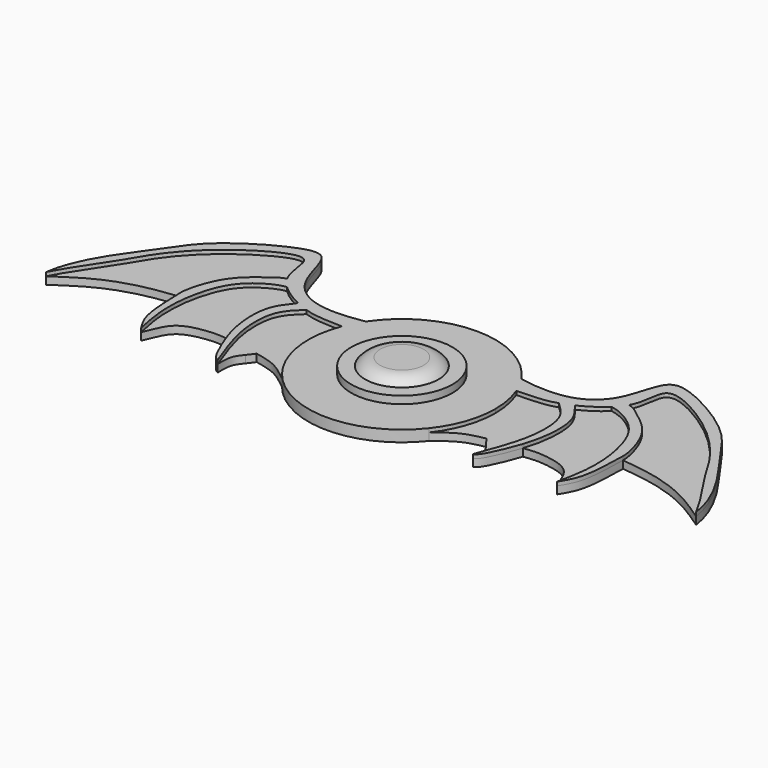
from build123d import *

# Parameters (mm, degrees)
F1_DEPTH = 3
F2_R     = 13.5064277213
F3_DEPTH = 5
F4_R     = 9.8042212389
F5_DEPTH = 7
F7_DEPTH = 2
F8_DEPTH = 3


# Not quite as in the source:
# - a fillet or chamfer that OpenCascade refuses, or shapes differently, is made with other operations: its cross-section is extruded or revolved along the edge and cut away or added


with BuildPart() as f1:
    # F0 (on Top) → F1 (new body)
    with BuildSketch(Plane.XY):
        with BuildLine():
            ThreePointArc((-19.6218875172, -15.4913372651), (0, -25), (19.6218875172, -15.4913372651))
            add(Edge.make_bspline(
                [(20.7636337812, 13.92377507), (18.884492427, 12.8973675107), (13.2694896297, 9.830391573), (17.0839746859, -5.3747888898), (19.6218875172, -15.4913372651)],
                knots=[0, 0, 0, 0, 0.3346643665, 1, 1, 1, 1], degree=3))
            ThreePointArc((20.7636337812, 13.92377507), (0, 25), (-20.7636337812, 13.92377507))
            add(Edge.make_bspline(
                [(-20.7636337812, 13.92377507), (-18.884492427, 12.8973675107), (-13.2694896297, 9.830391573), (-17.0839746859, -5.3747888898), (-19.6218875172, -15.4913372651)],
                knots=[0, 0, 0, 0, 0.3346643665, 1, 1, 1, 1], degree=3))
        make_face()
        with BuildLine():
            ThreePointArc((19.6218875172, -15.4913372651), (23.61723087, -8.1991710578), (25, 0))
            ThreePointArc((25, 0), (24.5689951544, 4.6221723357), (23.2908418319, 9.0849703775))
            ThreePointArc((23.2908418319, 9.0849703775), (22.1597092287, 11.5735598197), (20.7636337812, 13.92377507))
            add(Edge.make_bspline(
                [(20.7636337812, 13.92377507), (18.884492427, 12.8973675107), (13.2694896297, 9.830391573), (17.0839746859, -5.3747888898), (19.6218875172, -15.4913372651)],
                knots=[0, 0, 0, 0, 0.3346643665, 1, 1, 1, 1], degree=3))
        make_face()
        with BuildLine():
            ThreePointArc((-23.2908418319, 9.0849703775), (-24.7259844978, -3.6912993126), (-19.6218875172, -15.4913372651))
            add(Edge.make_bspline(
                [(-20.7636337812, 13.92377507), (-18.884492427, 12.8973675107), (-13.2694896297, 9.830391573), (-17.0839746859, -5.3747888898), (-19.6218875172, -15.4913372651)],
                knots=[0, 0, 0, 0, 0.3346643665, 1, 1, 1, 1], degree=3))
            ThreePointArc((-20.7636337812, 13.92377507), (-22.1597092287, 11.5735598197), (-23.2908418319, 9.0849703775))
        make_face()
    extrude(amount=F1_DEPTH)

    # F2 (on Top) → F3 (join)
    with BuildSketch(Plane.XY):
        Circle(F2_R)
    extrude(amount=F3_DEPTH)

    # F4 (on Top) → F5 (join)
    with BuildSketch(Plane.XY):
        Circle(F4_R)
    extrude(amount=F5_DEPTH)

    # F6: fillet of radius 5 on 1 edges, made by hand

    # F6_s1 → F6_t2 (revolve, cut)
    with BuildSketch(Plane.XZ):
        with BuildLine():
            ThreePointArc((9.8042212389, 5), (8.0402892164, 6.472135955), (5.8042212389, 7))
            Line((5.8042212389, 7), (9.8042212389, 7))
            Line((9.8042212389, 7), (9.8042212389, 5))
        make_face()
    revolve(axis=Axis((0, 0, 7), (0, 0, 1)), mode=Mode.SUBTRACT)

    # F0 (on Top) → F7 (join)
    with BuildSketch(Plane.XY):
        with BuildLine():
            ThreePointArc((20.7636337812, 13.92377507), (22.1597092287, 11.5735598197), (23.2908418319, 9.0849703775))
            add(Edge.make_bspline(
                [(23.2908418319, 9.0849703775), (27.8215143515, 9.3257680742), (30.2320226011, 9.1590800923), (33.7177366018, 10.2821364999)],
                knots=[0, 0, 0, 0, 0.1231403921, 0.1231403921, 0.1231403921, 0.1231403921], degree=3))
            add(Edge.make_bspline(
                [(33.7177366018, 10.2821364999), (34.7454077104, 10.6132401484), (35.866536795, 11.0564496893), (37.004531993, 11.5978625395)],
                knots=[0.1231403921, 0.1231403921, 0.1231403921, 0.1231403921, 0.1594450984, 0.1594450984, 0.1594450984, 0.1594450984], degree=3))
            add(Edge.make_bspline(
                [(37.004531993, 11.5978625395), (39.2474500295, 12.6649537267), (41.555886116, 14.1135251746), (43.3434300018, 15.8371345407)],
                knots=[0.1594450984, 0.1594450984, 0.1594450984, 0.1594450984, 0.2309994255, 0.2309994255, 0.2309994255, 0.2309994255], degree=3))
            add(Edge.make_bspline(
                [(43.3434300018, 15.8371345407), (44.2810928585, 16.7412603051), (45.0754287668, 17.7210645793), (45.641798526, 18.7611840665)],
                knots=[0.2309994255, 0.2309994255, 0.2309994255, 0.2309994255, 0.2685335165, 0.2685335165, 0.2685335165, 0.2685335165], degree=3))
            add(Edge.make_bspline(
                [(45.641798526, 18.7611840665), (47.3352689159, 21.8711868955), (46.777744727, 27.7747473366), (51.8560066338, 29.065553317), (66.3600577374, 20.2512677808), (74.7298542288, 9.6960609054), (77.7930462557, 3.5527051654), (84.7415977894, -6.1442317778), (86.8003591895, -10.2821364999)],
                knots=[0.2685335165, 0.2685335165, 0.2685335165, 0.2685335165, 0.3807620926, 0.4500912377, 0.6051903106, 0.7450551623, 0.8470726585, 1, 1, 1, 1], degree=3))
            add(Edge.make_bspline(
                [(20.7636337812, 13.92377507), (25.353260156, 13.083604301), (34.3722799665, 12.4739559617), (43.1666874947, 19.3658325346), (44.7883389447, 31.8865702273), (51.6235191398, 32.3410311281), (68.757647719, 22.5890249267), (75.2339965242, 11.4273433149), (85.5971213344, -1.5157287213), (86.8003591895, -10.2821364999)],
                knots=[0, 0, 0, 0, 0.1438051462, 0.2702269745, 0.4006587664, 0.4888335416, 0.6586500337, 0.8053535671, 1, 1, 1, 1], degree=3))
        make_face()
        with BuildLine():
            ThreePointArc((19.6218875172, -15.4913372651), (23.61723087, -8.1991710578), (25, 0))
            ThreePointArc((25, 0), (24.5689951544, 4.6221723357), (23.2908418319, 9.0849703775))
            ThreePointArc((23.2908418319, 9.0849703775), (22.1597092287, 11.5735598197), (20.7636337812, 13.92377507))
            add(Edge.make_bspline(
                [(20.7636337812, 13.92377507), (18.884492427, 12.8973675107), (13.2694896297, 9.830391573), (17.0839746859, -5.3747888898), (19.6218875172, -15.4913372651)],
                knots=[0, 0, 0, 0, 0.3346643665, 1, 1, 1, 1], degree=3))
        make_face()
        with BuildLine():
            ThreePointArc((23.2908418319, 9.0849703775), (24.5689951544, 4.6221723357), (25, 0))
            ThreePointArc((25, 0), (23.61723087, -8.1991710578), (19.6218875172, -15.4913372651))
            add(Edge.make_bspline(
                [(19.6218875172, -15.4913372651), (21.4152102231, -14.0609489213), (24.8604058768, -11.2746200768), (28.7928801922, -10.5001506768), (30.6888949126, -10.1227229461)],
                knots=[0, 0, 0, 0, 0.5172233423, 1, 1, 1, 1], degree=3))
            add(Edge.make_bspline(
                [(32.1116161516, -12.0142660523), (31.6373757386, -11.3837516835), (31.1631353256, -10.7532373148), (30.6888949126, -10.1227229461)],
                knots=[0, 0, 0, 0, 2.3668694612, 2.3668694612, 2.3668694612, 2.3668694612], degree=3))
            add(Edge.make_bspline(
                [(32.1116161516, -12.0142660523), (32.776720922, -12.8822985255), (34.1447409362, -14.3321949992), (34.1047637318, -17.2769145921), (34.0780636316, -18.8904348761)],
                knots=[0, 0, 0, 0, 0.4499025437, 1, 1, 1, 1], degree=3))
            add(Edge.make_bspline(
                [(33.7177366018, 10.2821364999), (35.3645415529, 8.7757476619), (38.884943387, 5.4848056386), (38.8140830901, -4.1284440887), (37.0736184249, -10.5819579136), (35.282158389, -15.8523198225), (34.0780636316, -18.8904348761)],
                knots=[0, 0, 0, 0, 0.2318500383, 0.4998701646, 0.7334854658, 1, 1, 1, 1], degree=3))
            add(Edge.make_bspline(
                [(23.2908418319, 9.0849703775), (27.8215143515, 9.3257680742), (30.2320226011, 9.1590800923), (33.7177366018, 10.2821364999)],
                knots=[0, 0, 0, 0, 0.1231403921, 0.1231403921, 0.1231403921, 0.1231403921], degree=3))
        make_face()
        with BuildLine():
            add(Edge.make_bspline(
                [(33.7177366018, 10.2821364999), (34.7454077104, 10.6132401484), (35.866536795, 11.0564496893), (37.004531993, 11.5978625395)],
                knots=[0.1231403921, 0.1231403921, 0.1231403921, 0.1231403921, 0.1594450984, 0.1594450984, 0.1594450984, 0.1594450984], degree=3))
            add(Edge.make_bspline(
                [(33.7177366018, 10.2821364999), (35.3645415529, 8.7757476619), (38.884943387, 5.4848056386), (38.8140830901, -4.1284440887), (37.0736184249, -10.5819579136), (35.282158389, -15.8523198225), (34.0780636316, -18.8904348761)],
                knots=[0, 0, 0, 0, 0.2318500383, 0.4998701646, 0.7334854658, 1, 1, 1, 1], degree=3))
            add(Edge.make_bspline(
                [(39.3599004471, -8.7854920866), (38.7249404903, -10.7452749087), (37.0180617267, -14.9012626381), (35.2493275964, -18.5335928874), (34.0780636316, -18.8904348761)],
                knots=[0.6277129418, 0.6277129418, 0.6277129418, 0.6277129418, 0.792816444, 1, 1, 1, 1], degree=3))
            add(Edge.make_bspline(
                [(37.004531993, 11.5978625395), (38.0800679502, 10.0046793736), (41.3336069296, 6.7268291074), (41.1834657071, -2.2502985215), (39.8295408824, -7.3359624778), (39.3599004471, -8.7854920866)],
                knots=[0, 0, 0, 0, 0.2173363693, 0.5055961378, 0.6277129418, 0.6277129418, 0.6277129418, 0.6277129418], degree=3))
        make_face()
        with BuildLine():
            add(Edge.make_bspline(
                [(37.004531993, 11.5978625395), (39.2474500295, 12.6649537267), (41.555886116, 14.1135251746), (43.3434300018, 15.8371345407)],
                knots=[0.1594450984, 0.1594450984, 0.1594450984, 0.1594450984, 0.2309994255, 0.2309994255, 0.2309994255, 0.2309994255], degree=3))
            add(Edge.make_bspline(
                [(37.004531993, 11.5978625395), (38.0800679502, 10.0046793736), (41.3336069296, 6.7268291074), (41.1834657071, -2.2502985215), (39.8295408824, -7.3359624778), (39.3599004471, -8.7854920866)],
                knots=[0, 0, 0, 0, 0.2173363693, 0.5055961378, 0.6277129418, 0.6277129418, 0.6277129418, 0.6277129418], degree=3))
            add(Edge.make_bspline(
                [(55.5573105812, -17.6151320338), (54.4439075888, -14.9875635555), (52.9703835571, -10.411043477), (46.6717355198, -8.6507292972), (42.2245726074, -8.3797506367), (40.2332096515, -8.6600986878), (39.3599004471, -8.7854920866)],
                knots=[0, 0, 0, 0, 0.3047383368, 0.5764576192, 0.8133522424, 1, 1, 1, 1], degree=3))
            add(Edge.make_bspline(
                [(43.3434300018, 15.8371345407), (45.3565623966, 15.5676262825), (49.9854795603, 13.2408710445), (54.5376514308, 8.1613285539), (57.1013516863, -1.3778788699), (57.1238501467, -10.2186225385), (56.0702038202, -15.2273425566), (55.5573105812, -17.6151320338)],
                knots=[0, 0, 0, 0, 0.1860076727, 0.3714288806, 0.5926344587, 0.8055769314, 1, 1, 1, 1], degree=3))
        make_face()
        with BuildLine():
            add(Edge.make_bspline(
                [(45.641798526, 18.7611840665), (47.0236524725, 18.4958354205), (50.5733406235, 15.7663353525), (56.3104736797, 11.1079119823), (58.8622688049, 3.2726876511), (59.0809752339, 0.6245344364), (59.0938226065, 0)],
                knots=[0, 0, 0, 0, 0.146943127, 0.3231645985, 0.5131967694, 0.5724247553, 0.5724247553, 0.5724247553, 0.5724247553], degree=3))
            add(Edge.make_bspline(
                [(43.3434300018, 15.8371345407), (44.2810928585, 16.7412603051), (45.0754287668, 17.7210645793), (45.641798526, 18.7611840665)],
                knots=[0.2309994255, 0.2309994255, 0.2309994255, 0.2309994255, 0.2685335165, 0.2685335165, 0.2685335165, 0.2685335165], degree=3))
            add(Edge.make_bspline(
                [(43.3434300018, 15.8371345407), (45.3565623966, 15.5676262825), (49.9854795603, 13.2408710445), (54.5376514308, 8.1613285539), (57.1013516863, -1.3778788699), (57.1238501467, -10.2186225385), (56.0702038202, -15.2273425566), (55.5573105812, -17.6151320338)],
                knots=[0, 0, 0, 0, 0.1860076727, 0.3714288806, 0.5926344587, 0.8055769314, 1, 1, 1, 1], degree=3))
            add(Edge.make_bspline(
                [(59.0938226065, 0), (59.1104927586, -0.8103667818), (58.9358631638, -3.6588287886), (58.782367202, -12.4944121501), (56.5431938855, -16.0569735079), (55.5573105812, -17.6151320338)],
                knots=[0.5724247553, 0.5724247553, 0.5724247553, 0.5724247553, 0.6492762299, 0.8452276156, 1, 1, 1, 1], degree=3))
        make_face()
        with BuildLine():
            add(Edge.make_bspline(
                [(59.0938226065, 0), (62.0265888913, -0.341290779), (68.0943487487, -1.0474058551), (78.0033682979, -4.2880779786), (83.850491985, -8.272167765), (86.8003591895, -10.2821364999)],
                knots=[0, 0, 0, 0, 0.3167243267, 0.6552882052, 1, 1, 1, 1], degree=3))
            add(Edge.make_bspline(
                [(45.641798526, 18.7611840665), (47.3352689159, 21.8711868955), (46.777744727, 27.7747473366), (51.8560066338, 29.065553317), (66.3600577374, 20.2512677808), (74.7298542288, 9.6960609054), (77.7930462557, 3.5527051654), (84.7415977894, -6.1442317778), (86.8003591895, -10.2821364999)],
                knots=[0.2685335165, 0.2685335165, 0.2685335165, 0.2685335165, 0.3807620926, 0.4500912377, 0.6051903106, 0.7450551623, 0.8470726585, 1, 1, 1, 1], degree=3))
            add(Edge.make_bspline(
                [(45.641798526, 18.7611840665), (47.0236524725, 18.4958354205), (50.5733406235, 15.7663353525), (56.3104736797, 11.1079119823), (58.8622688049, 3.2726876511), (59.0809752339, 0.6245344364), (59.0938226065, 0)],
                knots=[0, 0, 0, 0, 0.146943127, 0.3231645985, 0.5131967694, 0.5724247553, 0.5724247553, 0.5724247553, 0.5724247553], degree=3))
        make_face()
        with BuildLine():
            add(Edge.make_bspline(
                [(-19.6218875172, -15.4913372651), (-21.4152102231, -14.0609489213), (-24.8604058768, -11.2746200768), (-28.7928801922, -10.5001506768), (-30.6888949126, -10.1227229461)],
                knots=[0, 0, 0, 0, 0.5172233423, 1, 1, 1, 1], degree=3))
            ThreePointArc((-19.6218875172, -15.4913372651), (-24.7259844978, -3.6912993126), (-23.2908418319, 9.0849703775))
            add(Edge.make_bspline(
                [(-23.2908418319, 9.0849703775), (-27.8215143515, 9.3257680742), (-30.2320226011, 9.1590800923), (-33.7177366018, 10.2821364999)],
                knots=[0, 0, 0, 0, 0.1231403921, 0.1231403921, 0.1231403921, 0.1231403921], degree=3))
            add(Edge.make_bspline(
                [(-33.7177366018, 10.2821364999), (-35.3645415529, 8.7757476619), (-38.884943387, 5.4848056386), (-38.8140830901, -4.1284440887), (-37.0736184249, -10.5819579136), (-35.282158389, -15.8523198225), (-34.0780636316, -18.8904348761)],
                knots=[0, 0, 0, 0, 0.2318500383, 0.4998701646, 0.7334854658, 1, 1, 1, 1], degree=3))
            add(Edge.make_bspline(
                [(-32.1116161516, -12.0142660523), (-32.776720922, -12.8822985255), (-34.1447409362, -14.3321949992), (-34.1047637318, -17.2769145921), (-34.0780636316, -18.8904348761)],
                knots=[0, 0, 0, 0, 0.4499025437, 1, 1, 1, 1], degree=3))
            add(Edge.make_bspline(
                [(-32.1116161516, -12.0142660523), (-31.6373757386, -11.3837516835), (-31.1631353256, -10.7532373148), (-30.6888949126, -10.1227229461)],
                knots=[0, 0, 0, 0, 2.3668694612, 2.3668694612, 2.3668694612, 2.3668694612], degree=3))
        make_face()
        with BuildLine():
            add(Edge.make_bspline(
                [(-37.004531993, 11.5978625395), (-38.0800679502, 10.0046793736), (-41.3336069296, 6.7268291074), (-41.1834657071, -2.2502985215), (-39.8295408824, -7.3359624778), (-39.3599004471, -8.7854920866)],
                knots=[0, 0, 0, 0, 0.2173363693, 0.5055961378, 0.6277129418, 0.6277129418, 0.6277129418, 0.6277129418], degree=3))
            add(Edge.make_bspline(
                [(-37.004531993, 11.5978625395), (-39.2474500295, 12.6649537267), (-41.555886116, 14.1135251746), (-43.3434300018, 15.8371345407)],
                knots=[0.1594450984, 0.1594450984, 0.1594450984, 0.1594450984, 0.2309994255, 0.2309994255, 0.2309994255, 0.2309994255], degree=3))
            add(Edge.make_bspline(
                [(-43.3434300018, 15.8371345407), (-45.3565623966, 15.5676262825), (-49.9854795603, 13.2408710445), (-54.5376514308, 8.1613285539), (-57.1013516863, -1.3778788699), (-57.1238501467, -10.2186225385), (-56.0702038202, -15.2273425566), (-55.5573105812, -17.6151320338)],
                knots=[0, 0, 0, 0, 0.1860076727, 0.3714288806, 0.5926344587, 0.8055769314, 1, 1, 1, 1], degree=3))
            add(Edge.make_bspline(
                [(-55.5573105812, -17.6151320338), (-54.4439075888, -14.9875635555), (-52.9703835571, -10.411043477), (-46.6717355198, -8.6507292972), (-42.2245726074, -8.3797506367), (-40.2332096515, -8.6600986878), (-39.3599004471, -8.7854920866)],
                knots=[0, 0, 0, 0, 0.3047383368, 0.5764576192, 0.8133522424, 1, 1, 1, 1], degree=3))
        make_face()
        with BuildLine():
            add(Edge.make_bspline(
                [(-33.7177366018, 10.2821364999), (-35.3645415529, 8.7757476619), (-38.884943387, 5.4848056386), (-38.8140830901, -4.1284440887), (-37.0736184249, -10.5819579136), (-35.282158389, -15.8523198225), (-34.0780636316, -18.8904348761)],
                knots=[0, 0, 0, 0, 0.2318500383, 0.4998701646, 0.7334854658, 1, 1, 1, 1], degree=3))
            add(Edge.make_bspline(
                [(-33.7177366018, 10.2821364999), (-34.7454077104, 10.6132401484), (-35.866536795, 11.0564496893), (-37.004531993, 11.5978625395)],
                knots=[0.1231403921, 0.1231403921, 0.1231403921, 0.1231403921, 0.1594450984, 0.1594450984, 0.1594450984, 0.1594450984], degree=3))
            add(Edge.make_bspline(
                [(-37.004531993, 11.5978625395), (-38.0800679502, 10.0046793736), (-41.3336069296, 6.7268291074), (-41.1834657071, -2.2502985215), (-39.8295408824, -7.3359624778), (-39.3599004471, -8.7854920866)],
                knots=[0, 0, 0, 0, 0.2173363693, 0.5055961378, 0.6277129418, 0.6277129418, 0.6277129418, 0.6277129418], degree=3))
            add(Edge.make_bspline(
                [(-39.3599004471, -8.7854920866), (-38.7249404903, -10.7452749087), (-37.0180617267, -14.9012626381), (-35.2493275964, -18.5335928874), (-34.0780636316, -18.8904348761)],
                knots=[0.6277129418, 0.6277129418, 0.6277129418, 0.6277129418, 0.792816444, 1, 1, 1, 1], degree=3))
        make_face()
        with BuildLine():
            ThreePointArc((-23.2908418319, 9.0849703775), (-22.1597092287, 11.5735598197), (-20.7636337812, 13.92377507))
            add(Edge.make_bspline(
                [(-20.7636337812, 13.92377507), (-25.353260156, 13.083604301), (-34.3722799665, 12.4739559617), (-43.1666874947, 19.3658325346), (-44.7883389447, 31.8865702273), (-51.6235191398, 32.3410311281), (-68.757647719, 22.5890249267), (-75.2339965242, 11.4273433149), (-85.5971213344, -1.5157287213), (-86.8003591895, -10.2821364999)],
                knots=[0, 0, 0, 0, 0.1438051462, 0.2702269745, 0.4006587664, 0.4888335416, 0.6586500337, 0.8053535671, 1, 1, 1, 1], degree=3))
            add(Edge.make_bspline(
                [(-45.641798526, 18.7611840665), (-47.3352689159, 21.8711868955), (-46.777744727, 27.7747473366), (-51.8560066338, 29.065553317), (-66.3600577374, 20.2512677808), (-74.7298542288, 9.6960609054), (-77.7930462557, 3.5527051654), (-84.7415977894, -6.1442317778), (-86.8003591895, -10.2821364999)],
                knots=[0.2685335165, 0.2685335165, 0.2685335165, 0.2685335165, 0.3807620926, 0.4500912377, 0.6051903106, 0.7450551623, 0.8470726585, 1, 1, 1, 1], degree=3))
            add(Edge.make_bspline(
                [(-43.3434300018, 15.8371345407), (-44.2810928585, 16.7412603051), (-45.0754287668, 17.7210645793), (-45.641798526, 18.7611840665)],
                knots=[0.2309994255, 0.2309994255, 0.2309994255, 0.2309994255, 0.2685335165, 0.2685335165, 0.2685335165, 0.2685335165], degree=3))
            add(Edge.make_bspline(
                [(-37.004531993, 11.5978625395), (-39.2474500295, 12.6649537267), (-41.555886116, 14.1135251746), (-43.3434300018, 15.8371345407)],
                knots=[0.1594450984, 0.1594450984, 0.1594450984, 0.1594450984, 0.2309994255, 0.2309994255, 0.2309994255, 0.2309994255], degree=3))
            add(Edge.make_bspline(
                [(-33.7177366018, 10.2821364999), (-34.7454077104, 10.6132401484), (-35.866536795, 11.0564496893), (-37.004531993, 11.5978625395)],
                knots=[0.1231403921, 0.1231403921, 0.1231403921, 0.1231403921, 0.1594450984, 0.1594450984, 0.1594450984, 0.1594450984], degree=3))
            add(Edge.make_bspline(
                [(-23.2908418319, 9.0849703775), (-27.8215143515, 9.3257680742), (-30.2320226011, 9.1590800923), (-33.7177366018, 10.2821364999)],
                knots=[0, 0, 0, 0, 0.1231403921, 0.1231403921, 0.1231403921, 0.1231403921], degree=3))
        make_face()
        with BuildLine():
            add(Edge.make_bspline(
                [(-45.641798526, 18.7611840665), (-47.3352689159, 21.8711868955), (-46.777744727, 27.7747473366), (-51.8560066338, 29.065553317), (-66.3600577374, 20.2512677808), (-74.7298542288, 9.6960609054), (-77.7930462557, 3.5527051654), (-84.7415977894, -6.1442317778), (-86.8003591895, -10.2821364999)],
                knots=[0.2685335165, 0.2685335165, 0.2685335165, 0.2685335165, 0.3807620926, 0.4500912377, 0.6051903106, 0.7450551623, 0.8470726585, 1, 1, 1, 1], degree=3))
            add(Edge.make_bspline(
                [(-59.0938226065, 0), (-62.0265888913, -0.341290779), (-68.0943487487, -1.0474058551), (-78.0033682979, -4.2880779786), (-83.850491985, -8.272167765), (-86.8003591895, -10.2821364999)],
                knots=[0, 0, 0, 0, 0.3167243267, 0.6552882052, 1, 1, 1, 1], degree=3))
            add(Edge.make_bspline(
                [(-45.641798526, 18.7611840665), (-47.0236524725, 18.4958354205), (-50.5733406235, 15.7663353525), (-56.3104736797, 11.1079119823), (-58.8622688049, 3.2726876511), (-59.0809752339, 0.6245344364), (-59.0938226065, 0)],
                knots=[0, 0, 0, 0, 0.146943127, 0.3231645985, 0.5131967694, 0.5724247553, 0.5724247553, 0.5724247553, 0.5724247553], degree=3))
        make_face()
        with BuildLine():
            add(Edge.make_bspline(
                [(-43.3434300018, 15.8371345407), (-44.2810928585, 16.7412603051), (-45.0754287668, 17.7210645793), (-45.641798526, 18.7611840665)],
                knots=[0.2309994255, 0.2309994255, 0.2309994255, 0.2309994255, 0.2685335165, 0.2685335165, 0.2685335165, 0.2685335165], degree=3))
            add(Edge.make_bspline(
                [(-45.641798526, 18.7611840665), (-47.0236524725, 18.4958354205), (-50.5733406235, 15.7663353525), (-56.3104736797, 11.1079119823), (-58.8622688049, 3.2726876511), (-59.0809752339, 0.6245344364), (-59.0938226065, 0)],
                knots=[0, 0, 0, 0, 0.146943127, 0.3231645985, 0.5131967694, 0.5724247553, 0.5724247553, 0.5724247553, 0.5724247553], degree=3))
            add(Edge.make_bspline(
                [(-59.0938226065, 0), (-59.1104927586, -0.8103667818), (-58.9358631638, -3.6588287886), (-58.782367202, -12.4944121501), (-56.5431938855, -16.0569735079), (-55.5573105812, -17.6151320338)],
                knots=[0.5724247553, 0.5724247553, 0.5724247553, 0.5724247553, 0.6492762299, 0.8452276156, 1, 1, 1, 1], degree=3))
            add(Edge.make_bspline(
                [(-43.3434300018, 15.8371345407), (-45.3565623966, 15.5676262825), (-49.9854795603, 13.2408710445), (-54.5376514308, 8.1613285539), (-57.1013516863, -1.3778788699), (-57.1238501467, -10.2186225385), (-56.0702038202, -15.2273425566), (-55.5573105812, -17.6151320338)],
                knots=[0, 0, 0, 0, 0.1860076727, 0.3714288806, 0.5926344587, 0.8055769314, 1, 1, 1, 1], degree=3))
        make_face()
        with BuildLine():
            ThreePointArc((-23.2908418319, 9.0849703775), (-24.7259844978, -3.6912993126), (-19.6218875172, -15.4913372651))
            add(Edge.make_bspline(
                [(-20.7636337812, 13.92377507), (-18.884492427, 12.8973675107), (-13.2694896297, 9.830391573), (-17.0839746859, -5.3747888898), (-19.6218875172, -15.4913372651)],
                knots=[0, 0, 0, 0, 0.3346643665, 1, 1, 1, 1], degree=3))
            ThreePointArc((-20.7636337812, 13.92377507), (-22.1597092287, 11.5735598197), (-23.2908418319, 9.0849703775))
        make_face()
    extrude(amount=F7_DEPTH)

    # F0 (on Top) → F8 (join)
    with BuildSketch(Plane.XY):
        with BuildLine():
            ThreePointArc((20.7636337812, 13.92377507), (22.1597092287, 11.5735598197), (23.2908418319, 9.0849703775))
            add(Edge.make_bspline(
                [(23.2908418319, 9.0849703775), (27.8215143515, 9.3257680742), (30.2320226011, 9.1590800923), (33.7177366018, 10.2821364999)],
                knots=[0, 0, 0, 0, 0.1231403921, 0.1231403921, 0.1231403921, 0.1231403921], degree=3))
            add(Edge.make_bspline(
                [(33.7177366018, 10.2821364999), (34.7454077104, 10.6132401484), (35.866536795, 11.0564496893), (37.004531993, 11.5978625395)],
                knots=[0.1231403921, 0.1231403921, 0.1231403921, 0.1231403921, 0.1594450984, 0.1594450984, 0.1594450984, 0.1594450984], degree=3))
            add(Edge.make_bspline(
                [(37.004531993, 11.5978625395), (39.2474500295, 12.6649537267), (41.555886116, 14.1135251746), (43.3434300018, 15.8371345407)],
                knots=[0.1594450984, 0.1594450984, 0.1594450984, 0.1594450984, 0.2309994255, 0.2309994255, 0.2309994255, 0.2309994255], degree=3))
            add(Edge.make_bspline(
                [(43.3434300018, 15.8371345407), (44.2810928585, 16.7412603051), (45.0754287668, 17.7210645793), (45.641798526, 18.7611840665)],
                knots=[0.2309994255, 0.2309994255, 0.2309994255, 0.2309994255, 0.2685335165, 0.2685335165, 0.2685335165, 0.2685335165], degree=3))
            add(Edge.make_bspline(
                [(45.641798526, 18.7611840665), (47.3352689159, 21.8711868955), (46.777744727, 27.7747473366), (51.8560066338, 29.065553317), (66.3600577374, 20.2512677808), (74.7298542288, 9.6960609054), (77.7930462557, 3.5527051654), (84.7415977894, -6.1442317778), (86.8003591895, -10.2821364999)],
                knots=[0.2685335165, 0.2685335165, 0.2685335165, 0.2685335165, 0.3807620926, 0.4500912377, 0.6051903106, 0.7450551623, 0.8470726585, 1, 1, 1, 1], degree=3))
            add(Edge.make_bspline(
                [(20.7636337812, 13.92377507), (25.353260156, 13.083604301), (34.3722799665, 12.4739559617), (43.1666874947, 19.3658325346), (44.7883389447, 31.8865702273), (51.6235191398, 32.3410311281), (68.757647719, 22.5890249267), (75.2339965242, 11.4273433149), (85.5971213344, -1.5157287213), (86.8003591895, -10.2821364999)],
                knots=[0, 0, 0, 0, 0.1438051462, 0.2702269745, 0.4006587664, 0.4888335416, 0.6586500337, 0.8053535671, 1, 1, 1, 1], degree=3))
        make_face()
        with BuildLine():
            add(Edge.make_bspline(
                [(33.7177366018, 10.2821364999), (34.7454077104, 10.6132401484), (35.866536795, 11.0564496893), (37.004531993, 11.5978625395)],
                knots=[0.1231403921, 0.1231403921, 0.1231403921, 0.1231403921, 0.1594450984, 0.1594450984, 0.1594450984, 0.1594450984], degree=3))
            add(Edge.make_bspline(
                [(33.7177366018, 10.2821364999), (35.3645415529, 8.7757476619), (38.884943387, 5.4848056386), (38.8140830901, -4.1284440887), (37.0736184249, -10.5819579136), (35.282158389, -15.8523198225), (34.0780636316, -18.8904348761)],
                knots=[0, 0, 0, 0, 0.2318500383, 0.4998701646, 0.7334854658, 1, 1, 1, 1], degree=3))
            add(Edge.make_bspline(
                [(39.3599004471, -8.7854920866), (38.7249404903, -10.7452749087), (37.0180617267, -14.9012626381), (35.2493275964, -18.5335928874), (34.0780636316, -18.8904348761)],
                knots=[0.6277129418, 0.6277129418, 0.6277129418, 0.6277129418, 0.792816444, 1, 1, 1, 1], degree=3))
            add(Edge.make_bspline(
                [(37.004531993, 11.5978625395), (38.0800679502, 10.0046793736), (41.3336069296, 6.7268291074), (41.1834657071, -2.2502985215), (39.8295408824, -7.3359624778), (39.3599004471, -8.7854920866)],
                knots=[0, 0, 0, 0, 0.2173363693, 0.5055961378, 0.6277129418, 0.6277129418, 0.6277129418, 0.6277129418], degree=3))
        make_face()
        with BuildLine():
            add(Edge.make_bspline(
                [(45.641798526, 18.7611840665), (47.0236524725, 18.4958354205), (50.5733406235, 15.7663353525), (56.3104736797, 11.1079119823), (58.8622688049, 3.2726876511), (59.0809752339, 0.6245344364), (59.0938226065, 0)],
                knots=[0, 0, 0, 0, 0.146943127, 0.3231645985, 0.5131967694, 0.5724247553, 0.5724247553, 0.5724247553, 0.5724247553], degree=3))
            add(Edge.make_bspline(
                [(43.3434300018, 15.8371345407), (44.2810928585, 16.7412603051), (45.0754287668, 17.7210645793), (45.641798526, 18.7611840665)],
                knots=[0.2309994255, 0.2309994255, 0.2309994255, 0.2309994255, 0.2685335165, 0.2685335165, 0.2685335165, 0.2685335165], degree=3))
            add(Edge.make_bspline(
                [(43.3434300018, 15.8371345407), (45.3565623966, 15.5676262825), (49.9854795603, 13.2408710445), (54.5376514308, 8.1613285539), (57.1013516863, -1.3778788699), (57.1238501467, -10.2186225385), (56.0702038202, -15.2273425566), (55.5573105812, -17.6151320338)],
                knots=[0, 0, 0, 0, 0.1860076727, 0.3714288806, 0.5926344587, 0.8055769314, 1, 1, 1, 1], degree=3))
            add(Edge.make_bspline(
                [(59.0938226065, 0), (59.1104927586, -0.8103667818), (58.9358631638, -3.6588287886), (58.782367202, -12.4944121501), (56.5431938855, -16.0569735079), (55.5573105812, -17.6151320338)],
                knots=[0.5724247553, 0.5724247553, 0.5724247553, 0.5724247553, 0.6492762299, 0.8452276156, 1, 1, 1, 1], degree=3))
        make_face()
        with BuildLine():
            ThreePointArc((-23.2908418319, 9.0849703775), (-22.1597092287, 11.5735598197), (-20.7636337812, 13.92377507))
            add(Edge.make_bspline(
                [(-20.7636337812, 13.92377507), (-25.353260156, 13.083604301), (-34.3722799665, 12.4739559617), (-43.1666874947, 19.3658325346), (-44.7883389447, 31.8865702273), (-51.6235191398, 32.3410311281), (-68.757647719, 22.5890249267), (-75.2339965242, 11.4273433149), (-85.5971213344, -1.5157287213), (-86.8003591895, -10.2821364999)],
                knots=[0, 0, 0, 0, 0.1438051462, 0.2702269745, 0.4006587664, 0.4888335416, 0.6586500337, 0.8053535671, 1, 1, 1, 1], degree=3))
            add(Edge.make_bspline(
                [(-45.641798526, 18.7611840665), (-47.3352689159, 21.8711868955), (-46.777744727, 27.7747473366), (-51.8560066338, 29.065553317), (-66.3600577374, 20.2512677808), (-74.7298542288, 9.6960609054), (-77.7930462557, 3.5527051654), (-84.7415977894, -6.1442317778), (-86.8003591895, -10.2821364999)],
                knots=[0.2685335165, 0.2685335165, 0.2685335165, 0.2685335165, 0.3807620926, 0.4500912377, 0.6051903106, 0.7450551623, 0.8470726585, 1, 1, 1, 1], degree=3))
            add(Edge.make_bspline(
                [(-43.3434300018, 15.8371345407), (-44.2810928585, 16.7412603051), (-45.0754287668, 17.7210645793), (-45.641798526, 18.7611840665)],
                knots=[0.2309994255, 0.2309994255, 0.2309994255, 0.2309994255, 0.2685335165, 0.2685335165, 0.2685335165, 0.2685335165], degree=3))
            add(Edge.make_bspline(
                [(-37.004531993, 11.5978625395), (-39.2474500295, 12.6649537267), (-41.555886116, 14.1135251746), (-43.3434300018, 15.8371345407)],
                knots=[0.1594450984, 0.1594450984, 0.1594450984, 0.1594450984, 0.2309994255, 0.2309994255, 0.2309994255, 0.2309994255], degree=3))
            add(Edge.make_bspline(
                [(-33.7177366018, 10.2821364999), (-34.7454077104, 10.6132401484), (-35.866536795, 11.0564496893), (-37.004531993, 11.5978625395)],
                knots=[0.1231403921, 0.1231403921, 0.1231403921, 0.1231403921, 0.1594450984, 0.1594450984, 0.1594450984, 0.1594450984], degree=3))
            add(Edge.make_bspline(
                [(-23.2908418319, 9.0849703775), (-27.8215143515, 9.3257680742), (-30.2320226011, 9.1590800923), (-33.7177366018, 10.2821364999)],
                knots=[0, 0, 0, 0, 0.1231403921, 0.1231403921, 0.1231403921, 0.1231403921], degree=3))
        make_face()
        with BuildLine():
            add(Edge.make_bspline(
                [(-33.7177366018, 10.2821364999), (-35.3645415529, 8.7757476619), (-38.884943387, 5.4848056386), (-38.8140830901, -4.1284440887), (-37.0736184249, -10.5819579136), (-35.282158389, -15.8523198225), (-34.0780636316, -18.8904348761)],
                knots=[0, 0, 0, 0, 0.2318500383, 0.4998701646, 0.7334854658, 1, 1, 1, 1], degree=3))
            add(Edge.make_bspline(
                [(-33.7177366018, 10.2821364999), (-34.7454077104, 10.6132401484), (-35.866536795, 11.0564496893), (-37.004531993, 11.5978625395)],
                knots=[0.1231403921, 0.1231403921, 0.1231403921, 0.1231403921, 0.1594450984, 0.1594450984, 0.1594450984, 0.1594450984], degree=3))
            add(Edge.make_bspline(
                [(-37.004531993, 11.5978625395), (-38.0800679502, 10.0046793736), (-41.3336069296, 6.7268291074), (-41.1834657071, -2.2502985215), (-39.8295408824, -7.3359624778), (-39.3599004471, -8.7854920866)],
                knots=[0, 0, 0, 0, 0.2173363693, 0.5055961378, 0.6277129418, 0.6277129418, 0.6277129418, 0.6277129418], degree=3))
            add(Edge.make_bspline(
                [(-39.3599004471, -8.7854920866), (-38.7249404903, -10.7452749087), (-37.0180617267, -14.9012626381), (-35.2493275964, -18.5335928874), (-34.0780636316, -18.8904348761)],
                knots=[0.6277129418, 0.6277129418, 0.6277129418, 0.6277129418, 0.792816444, 1, 1, 1, 1], degree=3))
        make_face()
        with BuildLine():
            add(Edge.make_bspline(
                [(-43.3434300018, 15.8371345407), (-44.2810928585, 16.7412603051), (-45.0754287668, 17.7210645793), (-45.641798526, 18.7611840665)],
                knots=[0.2309994255, 0.2309994255, 0.2309994255, 0.2309994255, 0.2685335165, 0.2685335165, 0.2685335165, 0.2685335165], degree=3))
            add(Edge.make_bspline(
                [(-45.641798526, 18.7611840665), (-47.0236524725, 18.4958354205), (-50.5733406235, 15.7663353525), (-56.3104736797, 11.1079119823), (-58.8622688049, 3.2726876511), (-59.0809752339, 0.6245344364), (-59.0938226065, 0)],
                knots=[0, 0, 0, 0, 0.146943127, 0.3231645985, 0.5131967694, 0.5724247553, 0.5724247553, 0.5724247553, 0.5724247553], degree=3))
            add(Edge.make_bspline(
                [(-59.0938226065, 0), (-59.1104927586, -0.8103667818), (-58.9358631638, -3.6588287886), (-58.782367202, -12.4944121501), (-56.5431938855, -16.0569735079), (-55.5573105812, -17.6151320338)],
                knots=[0.5724247553, 0.5724247553, 0.5724247553, 0.5724247553, 0.6492762299, 0.8452276156, 1, 1, 1, 1], degree=3))
            add(Edge.make_bspline(
                [(-43.3434300018, 15.8371345407), (-45.3565623966, 15.5676262825), (-49.9854795603, 13.2408710445), (-54.5376514308, 8.1613285539), (-57.1013516863, -1.3778788699), (-57.1238501467, -10.2186225385), (-56.0702038202, -15.2273425566), (-55.5573105812, -17.6151320338)],
                knots=[0, 0, 0, 0, 0.1860076727, 0.3714288806, 0.5926344587, 0.8055769314, 1, 1, 1, 1], degree=3))
        make_face()
    extrude(amount=F8_DEPTH)


solid = f1.part
